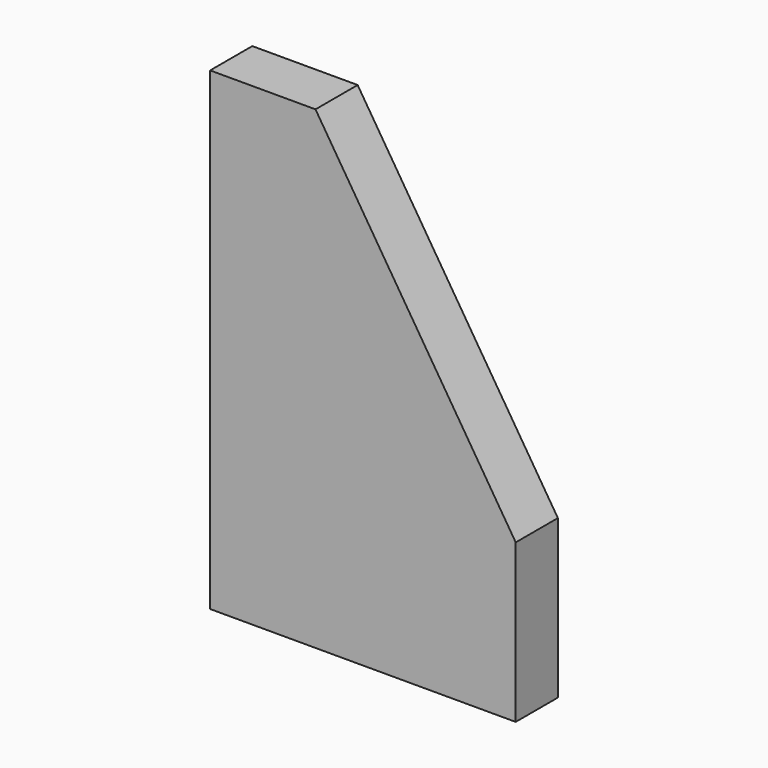
from build123d import *

# Parameters (mm, degrees)
F1_DEPTH = 5
F3_D     = 4.2
F3_DEPTH = 12.4
F3_TIP   = 1.2618073
F5_D     = 4.2
F5_DEPTH = 12.4
F5_TIP   = 1.2618073


# Not quite as in the source:
# - a feature names something its author has since deleted; it is built from what else it names


with BuildPart() as f1:
    # F0 (on Front) → F1 (new body, symmetric)
    with BuildSketch(Plane.XZ):
        Polygon((0, 90), (0, 0), (58, 0), (58, 30), (20, 90), align=None)
    extrude(amount=F1_DEPTH, both=True)

    # F3
    with Locations(Plane(origin=(0, 0, 0), x_dir=(1, 0, 0), z_dir=(0, 0, -1))):
        with Locations((26, 0), (48, 0)):
            Hole(F3_D / 2, depth=F3_DEPTH)
            with Locations((0, 0, -(F3_DEPTH + F3_TIP / 2))):  # 118° drill point
                Cone(0, F3_D / 2, F3_TIP, mode=Mode.SUBTRACT)

    # F5
    with Locations(Plane(origin=(0, 0, 0), x_dir=(0, -1, 0), z_dir=(-1, 0, 0))):
        with Locations((0, 20), (0, 82), (0, 51)):
            Hole(F5_D / 2, depth=F5_DEPTH)
            with Locations((0, 0, -(F5_DEPTH + F5_TIP / 2))):  # 118° drill point
                Cone(0, F5_D / 2, F5_TIP, mode=Mode.SUBTRACT)


solid = f1.part
